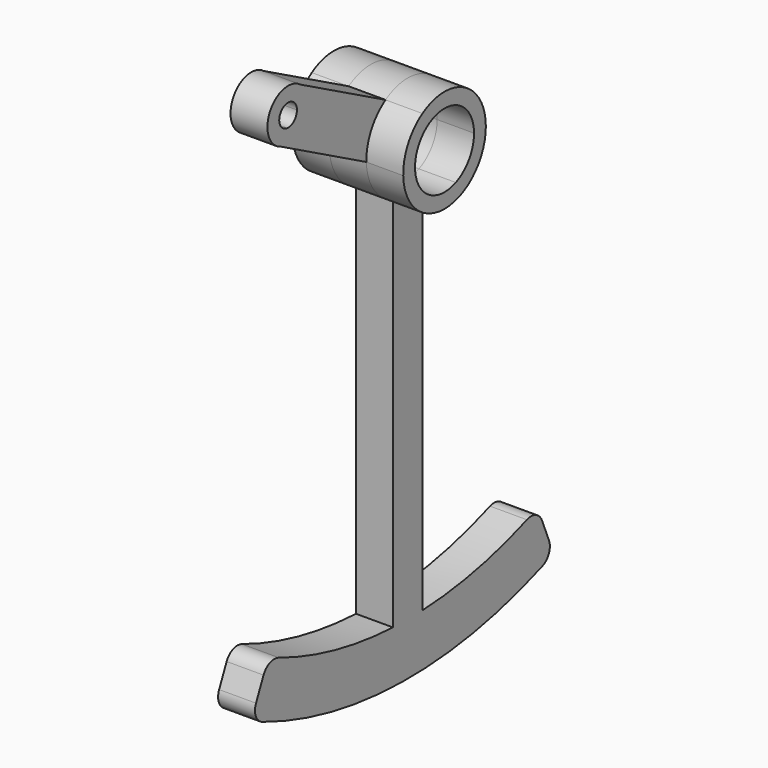
from build123d import *
from build123d import SkipClean  # not in build123d's __all__

# Parameters (mm, degrees)
F1_DEPTH      = 5
F2_DEPTH      = 10
F2_DEPTH_BACK = 5


with BuildPart() as f1:
    # F0 (on Right) → F1 (new body)
    with BuildSketch(Plane.YZ):
        with BuildLine():
            ThreePointArc((-2.0497591696, 58.6855219415), (-2.7158059717, 67.4442000024), (5, 63.2460578033))
            ThreePointArc((5, 63.2460578033), (4.1565190701, 60.4669663655), (1.9106603122, 58.6255191798))
            Line((1.9106603122, 58.6255191798), (2.6749244371, 56.7773037304))
            ThreePointArc((2.6749244371, 56.7773037304), (5.8191266982, 59.3553297904), (7, 63.2460578033))
            ThreePointArc((7, 63.2460578033), (3.3734494014, 69.3795591799), (-3.7485254675, 69.1577882453))
            ThreePointArc((-3.7485254675, 69.1577882453), (-6.1768933492, 66.539382651), (-6.9976278698, 63.0638376186))
            ThreePointArc((-6.9976278698, 63.0638376186), (-5.827409471, 59.3677464624), (-2.8696628374, 56.8613075968))
            Line((-2.8696628374, 56.8613075968), (-2.0497591696, 58.6855219415))
        make_face()
        with BuildLine():
            ThreePointArc((1.9106603122, 58.6255191798), (-0.0757443456, 58.2466315568), (-2.0497591696, 58.6855219415))
            Line((-2.0497591696, 58.6855219415), (-2.8696628374, 56.8613075968))
            ThreePointArc((-2.8696628374, 56.8613075968), (-2.6859296062, 56.7818654987), (-2.5, 56.707709388))
            Line((-2.5, 56.707709388), (2.5, 56.707709388))
            ThreePointArc((2.5, 56.707709388), (2.5876961907, 56.7419184733), (2.6749244371, 56.7773037304))
            Line((2.6749244371, 56.7773037304), (1.9106603122, 58.6255191798))
        make_face()
        with BuildLine():
            Line((-21.3842253571, 70.7343179555), (-6.9976278698, 63.0638376186))
            ThreePointArc((-6.9976278698, 63.0638376186), (-6.1768933492, 66.539382651), (-3.7485254675, 69.1577882453))
            Line((-3.7485254675, 69.1577882453), (-18.1351229548, 76.8282685822))
            ThreePointArc((-18.1351229548, 76.8282685822), (-17.1255151434, 75.5992014909), (-16.7640988794, 74.0502366327))
            ThreePointArc((-16.7640988794, 74.0502366327), (-18.2233199438, 71.2067842705), (-21.3842253571, 70.7343179555))
        make_face()
        with BuildLine():
            Line((2.5, 56.707709388), (-2.5, 56.707709388))
            ThreePointArc((-2.5, 56.707709388), (0, 56.2460578033), (2.5, 56.707709388))
        make_face()
        with BuildLine():
            ThreePointArc((2.5, 56.707709388), (0, 56.2460578033), (-2.5, 56.707709388))
            Line((-2.5, 56.707709388), (-2.5, 5.6896996604))
            ThreePointArc((-2.5, 5.6896996604), (0, 5.6354306355), (2.5, 5.6896996604))
            Line((2.5, 5.6896996604), (2.5, 56.707709388))
        make_face()
        with BuildLine():
            Line((-20.412130709, 72.5575589791), (-21.3842253571, 70.7343179555))
            ThreePointArc((-21.3842253571, 70.7343179555), (-18.2233199438, 71.2067842705), (-16.7640988794, 74.0502366327))
            ThreePointArc((-16.7640988794, 74.0502366327), (-17.1255151434, 75.5992014909), (-18.1351229548, 76.8282685822))
            Line((-18.1351229548, 76.8282685822), (-19.1072176029, 75.0050275585))
            ThreePointArc((-19.1072176029, 75.0050275585), (-18.8524824452, 74.5575225901), (-18.7640988794, 74.0502366327))
            ThreePointArc((-18.7640988794, 74.0502366327), (-19.2571350629, 72.9384705277), (-20.412130709, 72.5575589791))
        make_face()
        with BuildLine():
            ThreePointArc((-18.1351229548, 76.8282685822), (-23.352545554, 75.6968990565), (-21.3842253571, 70.7343179555))
            Line((-21.3842253571, 70.7343179555), (-20.412130709, 72.5575589791))
            ThreePointArc((-20.412130709, 72.5575589791), (-21.5877188828, 74.7559491), (-19.1072176029, 75.0050275585))
            Line((-19.1072176029, 75.0050275585), (-18.1351229548, 76.8282685822))
        make_face()
        with BuildLine():
            ThreePointArc((2.5, 5.6896996604), (0, 5.6354306355), (-2.5, 5.6896996604))
            ThreePointArc((-2.5, 5.6896996604), (-12.3544556578, 6.9757122555), (-21.8412756578, 9.9361802916))
            ThreePointArc((-21.8412756578, 9.9361802916), (-23.3409375081, 9.9429800309), (-24.4237277351, 8.9053879982))
            Line((-24.4237277351, 8.9053879982), (-25.6964663445, 6.0736552965))
            ThreePointArc((-25.6964663445, 6.0736552965), (-25.7303627866, 4.5138703516), (-24.6335625617, 3.4043175994))
            ThreePointArc((-24.6335625617, 3.4043175994), (-0.9803374174, -1.4600872963), (22.8093950074, 2.6855279633))
            ThreePointArc((22.8093950074, 2.6855279633), (23.939304908, 3.7613447039), (23.9526765567, 5.3214406119))
            Line((23.9526765567, 5.3214406119), (22.7663073553, 8.1904302912))
            ThreePointArc((22.7663073553, 8.1904302912), (21.7154471881, 9.260348424), (20.2162676541, 9.2989829539))
            ThreePointArc((20.2162676541, 9.2989829539), (11.5006058756, 6.7950132854), (2.5, 5.6896996604))
        make_face()
    extrude(amount=F1_DEPTH)

    # F0 (on Right) → F2 (join, two sides)
    with BuildSketch(Plane.YZ) as f2_sk:
        with BuildLine():
            ThreePointArc((1.9106603122, 58.6255191798), (-0.0757443456, 58.2466315568), (-2.0497591696, 58.6855219415))
            Line((-2.0497591696, 58.6855219415), (-2.8696628374, 56.8613075968))
            ThreePointArc((-2.8696628374, 56.8613075968), (-2.6859296062, 56.7818654987), (-2.5, 56.707709388))
            Line((-2.5, 56.707709388), (2.5, 56.707709388))
            ThreePointArc((2.5, 56.707709388), (2.5876961907, 56.7419184733), (2.6749244371, 56.7773037304))
            Line((2.6749244371, 56.7773037304), (1.9106603122, 58.6255191798))
        make_face()
        with BuildLine():
            ThreePointArc((-2.0497591696, 58.6855219415), (-2.7158059717, 67.4442000024), (5, 63.2460578033))
            ThreePointArc((5, 63.2460578033), (4.1565190701, 60.4669663655), (1.9106603122, 58.6255191798))
            Line((1.9106603122, 58.6255191798), (2.6749244371, 56.7773037304))
            ThreePointArc((2.6749244371, 56.7773037304), (5.8191266982, 59.3553297904), (7, 63.2460578033))
            ThreePointArc((7, 63.2460578033), (3.3734494014, 69.3795591799), (-3.7485254675, 69.1577882453))
            ThreePointArc((-3.7485254675, 69.1577882453), (-6.1768933492, 66.539382651), (-6.9976278698, 63.0638376186))
            ThreePointArc((-6.9976278698, 63.0638376186), (-5.827409471, 59.3677464624), (-2.8696628374, 56.8613075968))
            Line((-2.8696628374, 56.8613075968), (-2.0497591696, 58.6855219415))
        make_face()
        with BuildLine():
            Line((2.5, 56.707709388), (-2.5, 56.707709388))
            ThreePointArc((-2.5, 56.707709388), (0, 56.2460578033), (2.5, 56.707709388))
        make_face()
    with SkipClean():  # cleaning this boolean's faces spoils the solid; the shape is the same uncleaned
        extrude(amount=F2_DEPTH)
        extrude(f2_sk.sketch, amount=-F2_DEPTH_BACK)


solid = f1.part
